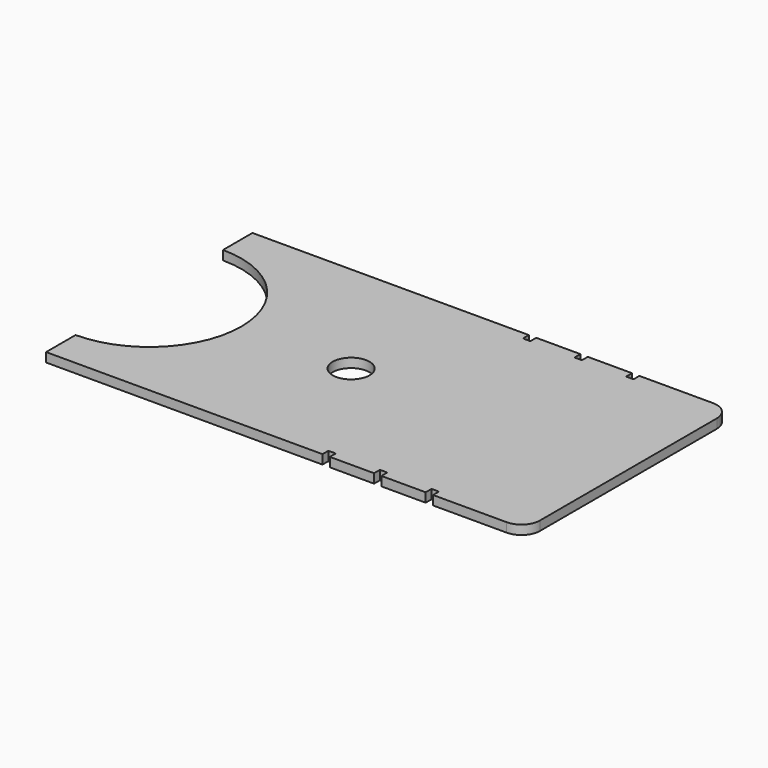
from build123d import *

# Parameters (mm, degrees)
F0_R     = 6.35
F1_DEPTH = 3.175


# Not quite as in the source:
# - a feature names something its author has since deleted; it is built from what else it names


with BuildPart() as f1:
    # F0 (on Top) → F1 (new body)
    with BuildSketch(Plane.XY):
        with BuildLine():
            Line((50.546, -43.7890713215), (75.946, -43.7890713215))
            ThreePointArc((75.946, -43.7890713215), (80.4361280605, -41.929199382), (82.296, -37.4390713215))
            Line((82.296, -37.4390713215), (82.296, 38.7609286785))
            ThreePointArc((82.296, 38.7609286785), (80.4361280605, 43.251056739), (75.946, 45.1109286785))
            Line((75.946, 45.1109286785), (50.546, 45.1109286785))
            Line((50.546, 45.1109286785), (50.546, 42.5709286785))
            Line((50.546, 42.5709286785), (48.006, 42.5709286785))
            Line((48.006, 42.5709286785), (48.006, 45.1109286785))
            Line((48.006, 45.1109286785), (32.766, 45.1109286785))
            Line((32.766, 45.1109286785), (32.766, 42.5709286785))
            Line((32.766, 42.5709286785), (30.226, 42.5709286785))
            Line((30.226, 42.5709286785), (30.226, 45.1109286785))
            Line((30.226, 45.1109286785), (14.986, 45.1109286785))
            Line((14.986, 45.1109286785), (14.986, 42.5709286785))
            Line((14.986, 42.5709286785), (12.446, 42.5709286785))
            Line((12.446, 42.5709286785), (12.446, 45.1109286785))
            Line((12.446, 45.1109286785), (-38.354, 45.1109286785))
            Line((-38.354, 45.1109286785), (-38.354, -43.7890713215))
            Line((-38.354, -43.7890713215), (12.446, -43.7890713215))
            Line((12.446, -43.7890713215), (12.446, -41.2490713215))
            Line((12.446, -41.2490713215), (14.986, -41.2490713215))
            Line((14.986, -41.2490713215), (14.986, -43.7890713215))
            Line((14.986, -43.7890713215), (30.226, -43.7890713215))
            Line((30.226, -43.7890713215), (30.226, -41.2490713215))
            Line((30.226, -41.2490713215), (32.766, -41.2490713215))
            Line((32.766, -41.2490713215), (32.766, -43.7890713215))
            Line((32.766, -43.7890713215), (48.006, -43.7890713215))
            Line((48.006, -43.7890713215), (48.006, -41.2490713215))
            Line((48.006, -41.2490713215), (50.546, -41.2490713215))
            Line((50.546, -41.2490713215), (50.546, -43.7890713215))
        make_face()
        with Locations((-12.7, 0)):
            Circle(F0_R, mode=Mode.SUBTRACT)
        with BuildLine():
            Line((-82.804, -43.7890713215), (-38.354, -43.7890713215))
            Line((-38.354, -43.7890713215), (-38.354, 45.1109286785))
            Line((-38.354, 45.1109286785), (-82.804, 45.1109286785))
            Line((-82.804, 45.1109286785), (-82.804, 32.4109286785))
            ThreePointArc((-82.804, 32.4109286785), (-51.054, 0.6609286785), (-82.804, -31.0890713215))
            Line((-82.804, -31.0890713215), (-82.804, -43.7890713215))
        make_face()
    extrude(amount=F1_DEPTH)


solid = f1.part
